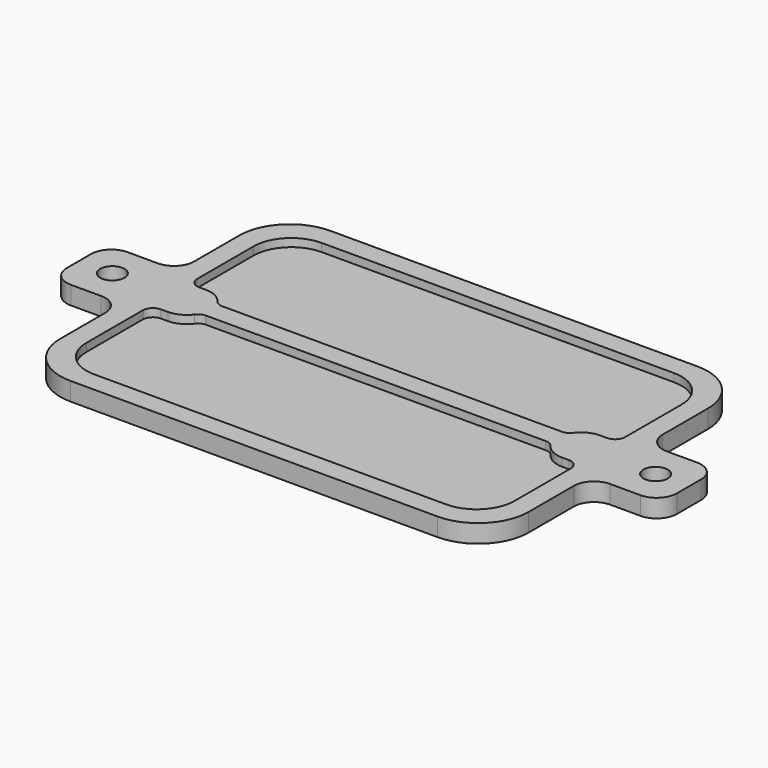
from build123d import *

# Parameters (mm, degrees)
F0_W      = 117.729
F0_H      = 81.661
F1_DEPTH  = 2.54
F2_W      = 117.729
F2_H      = 81.661
F3_DEPTH  = 2.032
F4_R      = 12.7
F5_W      = 17.78
F5_H      = 17.78
F6_DEPTH  = 4.572
F7_R      = 5.08
F13_R     = 3.048
F14_DEPTH = 4.573


# Not quite as in the source:
# - a feature of the source that left no trace in its solid (it failed there, or was rolled back) is left out
# - a pattern or mirror of a feature is missing from the dataset's text; its kind, count and spacing are read off the source's solid


with BuildPart() as f1:
    # F0 (on Top) → F1 (new body)
    with BuildSketch(Plane.XY):
        with Locations((-58.8645, 40.8305)):
            Rectangle(F0_W, F0_H)
    extrude(amount=F1_DEPTH)

    # F2 (on face) → F3 (join)
    with BuildSketch(Plane.XY.offset(2.54)):
        with Locations((-58.8645, 40.8305)):
            Rectangle(F2_W, F2_H)
        with BuildLine():
            ThreePointArc((-5.08, 14.605), (-7.8698079092, 7.8698079092), (-14.605, 5.08))
            Line((-14.605, 5.08), (-103.124, 5.08))
            ThreePointArc((-103.124, 5.08), (-109.8591920908, 7.8698079092), (-112.649, 14.605))
            Line((-112.649, 14.605), (-112.649, 32.2905))
            ThreePointArc((-112.649, 32.2905), (-111.9050512242, 34.0865512242), (-110.109, 34.8305))
            Line((-110.109, 34.8305), (-108.3945, 34.8305))
            ThreePointArc((-108.3945, 34.8305), (-105.6939926316, 35.4725843649), (-103.5714697827, 37.2614133489))
            ThreePointArc((-103.5714697827, 37.2614133489), (-102.67293511, 38.0186842855), (-101.529720324, 38.2905))
            Line((-101.529720324, 38.2905), (-58.8645, 38.2905))
            Line((-58.8645, 38.2905), (-16.199279676, 38.2905))
            ThreePointArc((-16.199279676, 38.2905), (-15.05606489, 38.0186842855), (-14.1575302173, 37.2614133489))
            ThreePointArc((-14.1575302173, 37.2614133489), (-12.0350073684, 35.4725843649), (-9.3345, 34.8305))
            Line((-9.3345, 34.8305), (-7.62, 34.8305))
            ThreePointArc((-7.62, 34.8305), (-5.8239487758, 34.0865512242), (-5.08, 32.2905))
            Line((-5.08, 32.2905), (-5.08, 14.605))
        make_face(mode=Mode.SUBTRACT)
        with BuildLine():
            Line((-103.124, 76.581), (-14.605, 76.581))
            ThreePointArc((-14.605, 76.581), (-7.8698079092, 73.7911920908), (-5.08, 67.056))
            Line((-5.08, 67.056), (-5.08, 49.3705))
            ThreePointArc((-5.08, 49.3705), (-5.8239487758, 47.5744487758), (-7.62, 46.8305))
            Line((-7.62, 46.8305), (-9.3345, 46.8305))
            ThreePointArc((-9.3345, 46.8305), (-12.0350073684, 46.1884156351), (-14.1575302173, 44.3995866511))
            ThreePointArc((-14.1575302173, 44.3995866511), (-15.05606489, 43.6423157145), (-16.199279676, 43.3705))
            Line((-16.199279676, 43.3705), (-58.8645, 43.3705))
            Line((-58.8645, 43.3705), (-101.529720324, 43.3705))
            ThreePointArc((-101.529720324, 43.3705), (-102.67293511, 43.6423157145), (-103.5714697827, 44.3995866511))
            ThreePointArc((-103.5714697827, 44.3995866511), (-105.6939926316, 46.1884156351), (-108.3945, 46.8305))
            Line((-108.3945, 46.8305), (-110.109, 46.8305))
            ThreePointArc((-110.109, 46.8305), (-111.9050512242, 47.5744487758), (-112.649, 49.3705))
            Line((-112.649, 49.3705), (-112.649, 67.056))
            ThreePointArc((-112.649, 67.056), (-109.8591920908, 73.7911920908), (-103.124, 76.581))
        make_face(mode=Mode.SUBTRACT)
    extrude(amount=F3_DEPTH)

    # F4
    f4_edges = [f1.edges().sort_by_distance(p)[0] for p in [
        (-117.729, 0, 2.286),
        (-117.729, 81.661, 2.286),
        (0, 81.661, 2.286),
        (0, 0, 2.286),
    ]]
    fillet(f4_edges, radius=F4_R)

    # F5 (on face) → F6 (join, through all)
    with BuildSketch(Plane.XY.offset(4.572)):
        with Locations((8.89, 40.8305)):
            Rectangle(F5_W, F5_H)
    f6 = extrude(amount=-F6_DEPTH)

    # F6_copies: F6 across plane
    add(f6.mirror(Plane(origin=(-58.8645, 0, 0), x_dir=(0, 0, -1), z_dir=(-1, 0, 0))))

    # F7
    f7_edges = [f1.edges().sort_by_distance(p)[0] for p in [
        (0, 31.9405, 2.286),
        (0, 49.7205, 2.286),
        (17.78, 49.7205, 2.286),
        (17.78, 31.9405, 2.286),
        (-117.729, 49.7205, 2.286),
        (-117.729, 31.9405, 2.286),
        (-135.509, 49.7205, 2.286),
        (-135.509, 31.9405, 2.286),
    ]]
    fillet(f7_edges, radius=F7_R)

    # F13 (on face) → F14 (cut, through all)
    with BuildSketch(Plane.XY.offset(4.572)):
        with Locations((9.398, 40.8305)):
            Circle(F13_R)
        with Locations((-127.127, 40.8305)):
            Circle(F13_R)
    extrude(amount=-F14_DEPTH, mode=Mode.SUBTRACT)


solid = f1.part
